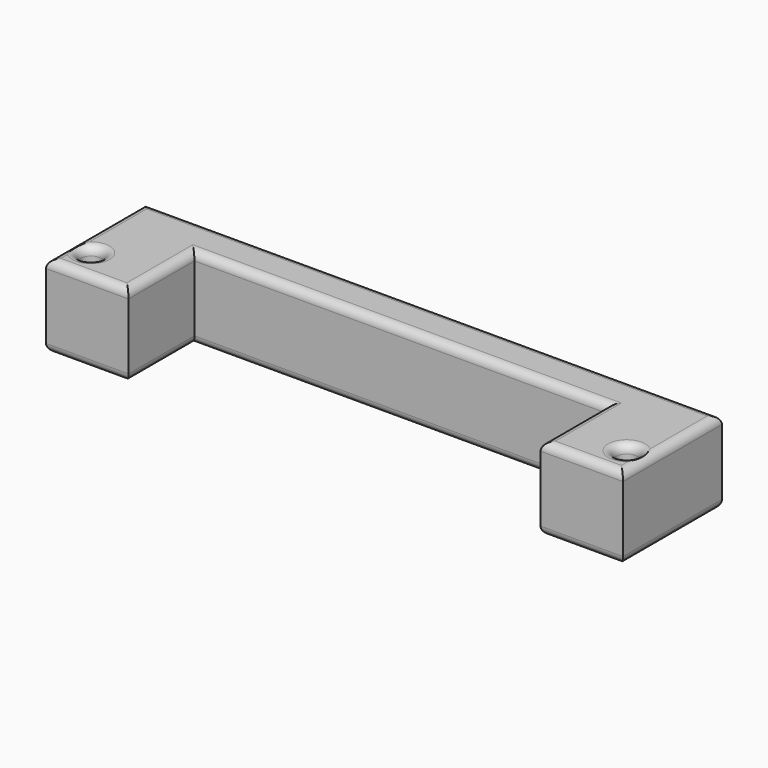
from build123d import *

# Parameters (mm, degrees)
F1_DEPTH     = 20
F3_D         = 5
F5_T1_DEPTH  = 150
F5_T3_DEPTH  = 40
F5_T5_DEPTH  = 30
F5_T7_DEPTH  = 25
F5_T9_DEPTH  = 100
F5_T11_DEPTH = 30
F5_T25_DEPTH = 105
F5_T29_DEPTH = 30
F5_T36_DEPTH = 30
F5_T40_DEPTH = 105
F5_T47_DEPTH = 30
F5_T51_DEPTH = 105
F5_T58_DEPTH = 105
F5_T62_DEPTH = 30


# Not quite as in the source:
# - a fillet or chamfer that OpenCascade refuses, or shapes differently, is made with other operations: its cross-section is extruded or revolved along the edge and cut away or added


with BuildPart() as f1:
    # F0 (on Top) → F1 (new body)
    with BuildSketch(Plane.XY):
        Polygon((70, 30), (0, 30), (0, 20), (50, 20), (50, 0), (70, 0), align=None)
    extrude(amount=F1_DEPTH)

    # F3 (through all)
    with Locations(Plane(origin=(0, 0, 0), x_dir=(1, 0, 0), z_dir=(0, 0, -1))):
        with Locations((65, -7.3669357225)):
            Hole(F3_D / 2)

    # F4: F1 across face


with BuildPart() as f1_1:
    add(f1.part)
    add(f1.part.mirror(Plane(origin=(0, 25, 10), x_dir=(0, -1, 0), z_dir=(-1, 0, 0))))

    # F5: fillet of radius 2 on 20 edges, made by hand

    # F5_s2 → F5_t1 (cut)
    with BuildSketch(Plane.YZ.offset(-75)):
        with BuildLine():
            ThreePointArc((30, 18), (29.4142135624, 19.4142135624), (28, 20))
            Line((28, 20), (30, 20))
            Line((30, 20), (30, 18))
        make_face()
        with BuildLine():
            ThreePointArc((30, 2), (29.4142135624, 0.5857864376), (28, 0))
            Line((28, 0), (30, 0))
            Line((30, 0), (30, 2))
        make_face()
    extrude(amount=F5_T1_DEPTH, mode=Mode.SUBTRACT)

    # F5_s4 → F5_t3 (cut)
    with BuildSketch(Plane.XZ.offset(-35)):
        with BuildLine():
            ThreePointArc((-70, 18), (-69.4142135624, 19.4142135624), (-68, 20))
            Line((-68, 20), (-70, 20))
            Line((-70, 20), (-70, 18))
        make_face()
        with BuildLine():
            ThreePointArc((68, 20), (69.4142135624, 19.4142135624), (70, 18))
            Line((70, 18), (70, 20))
            Line((70, 20), (68, 20))
        make_face()
        with BuildLine():
            ThreePointArc((-68, 0), (-69.4142135624, 0.5857864376), (-70, 2))
            Line((-70, 2), (-70, 0))
            Line((-70, 0), (-68, 0))
        make_face()
        with BuildLine():
            ThreePointArc((68, 0), (69.4142135624, 0.5857864376), (70, 2))
            Line((70, 2), (70, 0))
            Line((70, 0), (68, 0))
        make_face()
    extrude(amount=F5_T3_DEPTH, mode=Mode.SUBTRACT)

    # F5_s6 → F5_t5 (cut)
    with BuildSketch(Plane.YZ.offset(-75)):
        with BuildLine():
            ThreePointArc((0, 18), (0.5857864376, 19.4142135624), (2, 20))
            Line((2, 20), (0, 20))
            Line((0, 20), (0, 18))
        make_face()
        with BuildLine():
            ThreePointArc((2, 0), (0.5857864376, 0.5857864376), (0, 2))
            Line((0, 2), (0, 0))
            Line((0, 0), (2, 0))
        make_face()
    extrude(amount=F5_T5_DEPTH, mode=Mode.SUBTRACT)

    # F5_s8 → F5_t7 (cut)
    with BuildSketch(Plane.XZ.offset(-20)):
        with BuildLine():
            ThreePointArc((-50, 18), (-50.5857864376, 19.4142135624), (-52, 20))
            Line((-52, 20), (-50, 20))
            Line((-50, 20), (-50, 18))
        make_face()
        with BuildLine():
            ThreePointArc((50, 18), (50.5857864376, 19.4142135624), (52, 20))
            Line((52, 20), (50, 20))
            Line((50, 20), (50, 18))
        make_face()
        with BuildLine():
            ThreePointArc((-52, 0), (-50.5857864376, 0.5857864376), (-50, 2))
            Line((-50, 2), (-50, 0))
            Line((-50, 0), (-52, 0))
        make_face()
        with BuildLine():
            ThreePointArc((52, 0), (50.5857864376, 0.5857864376), (50, 2))
            Line((50, 2), (50, 0))
            Line((50, 0), (52, 0))
        make_face()
    extrude(amount=F5_T7_DEPTH, mode=Mode.SUBTRACT)

    # F5_s10 → F5_t9 (cut)
    with BuildSketch(Plane.YZ.offset(-50)):
        with BuildLine():
            ThreePointArc((20, 18), (20.5857864376, 19.4142135624), (22, 20))
            Line((22, 20), (20, 20))
            Line((20, 20), (20, 18))
        make_face()
        with BuildLine():
            ThreePointArc((22, 0), (20.5857864376, 0.5857864376), (20, 2))
            Line((20, 2), (20, 0))
            Line((20, 0), (22, 0))
        make_face()
    extrude(amount=F5_T9_DEPTH, mode=Mode.SUBTRACT)

    # F5_s12 → F5_t11 (cut)
    with BuildSketch(Plane.YZ.offset(45)):
        with BuildLine():
            ThreePointArc((0, 18), (0.5857864376, 19.4142135624), (2, 20))
            Line((2, 20), (0, 20))
            Line((0, 20), (0, 18))
        make_face()
        with BuildLine():
            ThreePointArc((2, 0), (0.5857864376, 0.5857864376), (0, 2))
            Line((0, 2), (0, 0))
            Line((0, 0), (2, 0))
        make_face()
    extrude(amount=F5_T11_DEPTH, mode=Mode.SUBTRACT)

    # F5_s13 → F5_t14 (revolve, cut)
    with BuildSketch(Plane.XZ.offset(-7.3669357225)):
        with BuildLine():
            ThreePointArc((67.5, 18), (68.0857864376, 19.4142135624), (69.5, 20))
            Line((69.5, 20), (67.5, 20))
            Line((67.5, 20), (67.5, 18))
        make_face()
    revolve(axis=Axis((65, 7.3669357225, 20), (0, 0, -1)), mode=Mode.SUBTRACT)

    # F5_s15 → F5_t16 (revolve, cut)
    with BuildSketch(Plane.XZ.offset(-7.3669357225)):
        with BuildLine():
            ThreePointArc((-67.5, 18), (-68.0857864376, 19.4142135624), (-69.5, 20))
            Line((-69.5, 20), (-67.5, 20))
            Line((-67.5, 20), (-67.5, 18))
        make_face()
    revolve(axis=Axis((-65, 7.3669357225, 20), (0, 0, 1)), mode=Mode.SUBTRACT)

    # F5_s17 → F5_t18 (revolve, cut)
    with BuildSketch(Plane.XZ.offset(-7.3669357225)):
        with BuildLine():
            ThreePointArc((69.5, 0), (68.0857864376, 0.5857864376), (67.5, 2))
            Line((67.5, 2), (67.5, 0))
            Line((67.5, 0), (69.5, 0))
        make_face()
    revolve(axis=Axis((65, 7.3669357225, 0), (0, 0, -1)), mode=Mode.SUBTRACT)

    # F5_s19 → F5_t20 (revolve, cut)
    with BuildSketch(Plane.XZ.offset(-7.3669357225)):
        with BuildLine():
            ThreePointArc((-69.5, 0), (-68.0857864376, 0.5857864376), (-67.5, 2))
            Line((-67.5, 2), (-67.5, 0))
            Line((-67.5, 0), (-69.5, 0))
        make_face()
    revolve(axis=Axis((-65, 7.3669357225, 0), (0, 0, 1)), mode=Mode.SUBTRACT)


with BuildPart() as f5_tool23:
    # F5_s24 → F5_t25 (new body)
    with BuildSketch(Plane.YZ.offset(-55)):
        with BuildLine():
            ThreePointArc((20, 18), (20.5857864376, 19.4142135624), (22, 20))
            Line((22, 20), (20, 20))
            Line((20, 20), (20, 18))
        make_face()
    extrude(amount=F5_T25_DEPTH)

    split(bisect_by=Plane.YZ.offset(-50), keep=Keep.BOTTOM)


with BuildPart() as f5_tool27:
    # F5_s28 → F5_t29 (new body)
    with BuildSketch(Plane.XZ.offset(-25)):
        with BuildLine():
            ThreePointArc((-50, 18), (-50.5857864376, 19.4142135624), (-52, 20))
            Line((-52, 20), (-50, 20))
            Line((-50, 20), (-50, 18))
        make_face()
    extrude(amount=F5_T29_DEPTH)

    split(bisect_by=Plane.XZ.offset(-20), keep=Keep.BOTTOM)


with BuildPart() as f5_tool23_1:
    add(f5_tool23.part)

    # F5_t31: intersect F5_tool27
    add(f5_tool27.part, mode=Mode.INTERSECT)


with BuildPart() as f1_2:
    add(f1_1.part)

    # F5_t21: cut F5_tool23
    add(f5_tool23_1.part, mode=Mode.SUBTRACT)


with BuildPart() as f5_tool34:
    # F5_s35 → F5_t36 (new body)
    with BuildSketch(Plane.XZ.offset(-25)):
        with BuildLine():
            ThreePointArc((50, 18), (50.5857864376, 19.4142135624), (52, 20))
            Line((52, 20), (50, 20))
            Line((50, 20), (50, 18))
        make_face()
    extrude(amount=F5_T36_DEPTH)

    split(bisect_by=Plane.XZ.offset(-20), keep=Keep.BOTTOM)


with BuildPart() as f5_tool38:
    # F5_s39 → F5_t40 (new body)
    with BuildSketch(Plane.YZ.offset(-50)):
        with BuildLine():
            ThreePointArc((20, 18), (20.5857864376, 19.4142135624), (22, 20))
            Line((22, 20), (20, 20))
            Line((20, 20), (20, 18))
        make_face()
    extrude(amount=F5_T40_DEPTH)

    split(bisect_by=Plane.YZ.offset(50), keep=Keep.TOP)


with BuildPart() as f5_tool34_1:
    add(f5_tool34.part)

    # F5_t42: intersect F5_tool38
    add(f5_tool38.part, mode=Mode.INTERSECT)


with BuildPart() as f1_3:
    add(f1_2.part)

    # F5_t32: cut F5_tool34
    add(f5_tool34_1.part, mode=Mode.SUBTRACT)


with BuildPart() as f5_tool45:
    # F5_s46 → F5_t47 (new body)
    with BuildSketch(Plane.XZ.offset(-25)):
        with BuildLine():
            ThreePointArc((-52, 0), (-50.5857864376, 0.5857864376), (-50, 2))
            Line((-50, 2), (-50, 0))
            Line((-50, 0), (-52, 0))
        make_face()
    extrude(amount=F5_T47_DEPTH)

    split(bisect_by=Plane.XZ.offset(-20), keep=Keep.BOTTOM)


with BuildPart() as f5_tool49:
    # F5_s50 → F5_t51 (new body)
    with BuildSketch(Plane.YZ.offset(50)):
        with BuildLine():
            ThreePointArc((22, 0), (20.5857864376, 0.5857864376), (20, 2))
            Line((20, 2), (20, 0))
            Line((20, 0), (22, 0))
        make_face()
    extrude(amount=-F5_T51_DEPTH)

    split(bisect_by=Plane.YZ.offset(-50), keep=Keep.BOTTOM)


with BuildPart() as f5_tool45_1:
    add(f5_tool45.part)

    # F5_t53: intersect F5_tool49
    add(f5_tool49.part, mode=Mode.INTERSECT)


with BuildPart() as f1_4:
    add(f1_3.part)

    # F5_t43: cut F5_tool45
    add(f5_tool45_1.part, mode=Mode.SUBTRACT)


with BuildPart() as f5_tool56:
    # F5_s57 → F5_t58 (new body)
    with BuildSketch(Plane.YZ.offset(55)):
        with BuildLine():
            ThreePointArc((22, 0), (20.5857864376, 0.5857864376), (20, 2))
            Line((20, 2), (20, 0))
            Line((20, 0), (22, 0))
        make_face()
    extrude(amount=-F5_T58_DEPTH)

    split(bisect_by=Plane.YZ.offset(50), keep=Keep.TOP)


with BuildPart() as f5_tool60:
    # F5_s61 → F5_t62 (new body)
    with BuildSketch(Plane.XZ.offset(-25)):
        with BuildLine():
            ThreePointArc((52, 0), (50.5857864376, 0.5857864376), (50, 2))
            Line((50, 2), (50, 0))
            Line((50, 0), (52, 0))
        make_face()
    extrude(amount=F5_T62_DEPTH)

    split(bisect_by=Plane.XZ.offset(-20), keep=Keep.BOTTOM)


with BuildPart() as f5_tool56_1:
    add(f5_tool56.part)

    # F5_t64: intersect F5_tool60
    add(f5_tool60.part, mode=Mode.INTERSECT)


with BuildPart() as f1_5:
    add(f1_4.part)

    # F5_t54: cut F5_tool56
    add(f5_tool56_1.part, mode=Mode.SUBTRACT)


solid = f1_5.part
